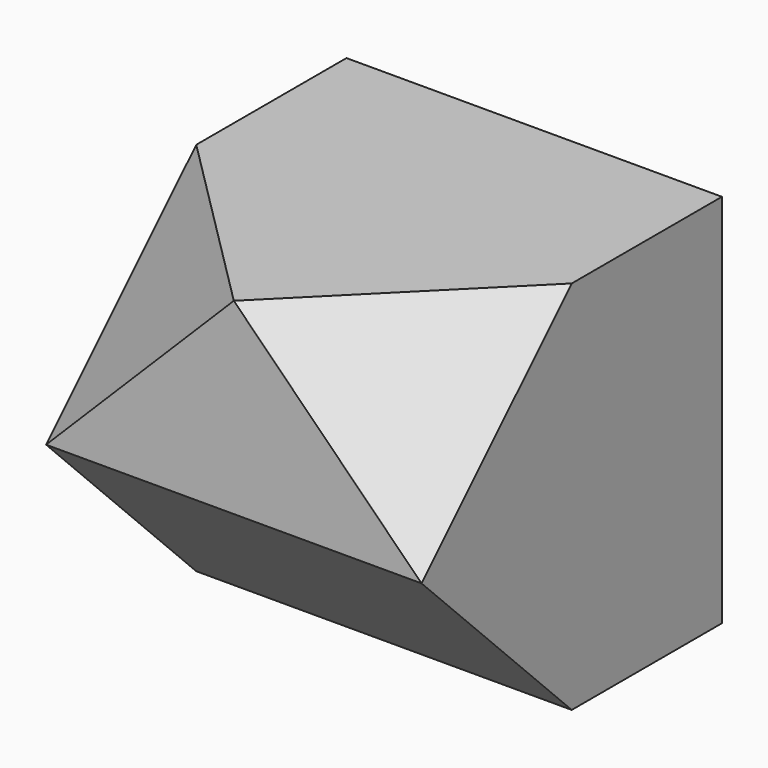
from build123d import *

# Parameters (mm, degrees)
F0_W     = 10
F0_H     = 5
F1_DEPTH = 5
F6_DEPTH = 2.8877513459


# Not quite as in the source:
# - a pattern or mirror of a feature is missing from the dataset's text; its kind, count and spacing are read off the source's solid


with BuildPart() as f1:
    # F0 (on Right) → F1 (new body, symmetric)
    with BuildSketch(Plane.YZ):
        with Locations((5, 2.5)):
            Rectangle(F0_W, F0_H)
        Polygon((10, 0), (0, 0), (5, -5), (10, -5), align=None)
    extrude(amount=F1_DEPTH, both=True)

    # F5 (on 3pt) → F6 (cut, through all)
    with BuildSketch(Plane(origin=(1.6666666667, -1.6666666667, 1.6666666667), x_dir=(0.8164965809, 0.4082482905, -0.4082482905), z_dir=(-0.5773502692, 0.5773502692, -0.5773502692))):
        Polygon((4.0824829046, 0), (-2.0412414523, -3.5355339059), (4.0824829046, -7.0710678119), align=None)
    f6 = extrude(amount=-F6_DEPTH, mode=Mode.SUBTRACT)

    # F6_copies: F6 across plane
    add(f6.mirror(Plane(origin=(0, 0, 0), x_dir=(0, 0, -1), z_dir=(-1, 0, 0))), mode=Mode.SUBTRACT)


solid = f1.part
